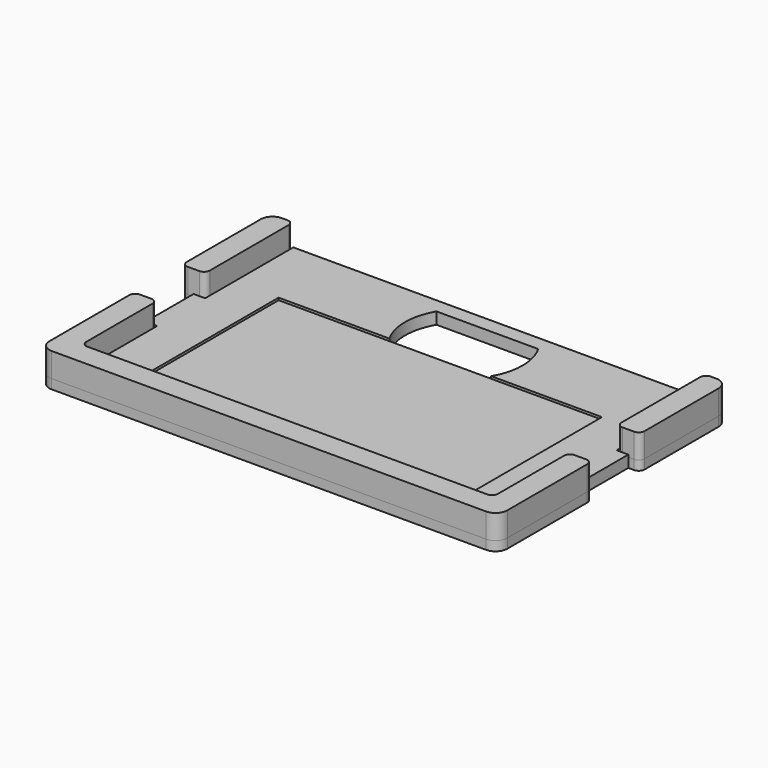
from build123d import *

# Parameters (mm, degrees)
F0_R     = 1.25
F0_W     = 2.5
F0_H     = 12.954
F0_W_2   = 69.85
F0_H_2   = 41.275
F1_DEPTH = 2.54
F2_DEPTH = 4.7625
F3_DEPTH = 0.5
F4_DEPTH = 0.5
F5_DEPTH = 3
F6_R     = 2.54
F6_2_R   = 2.54
F6_3_R   = 2.54
F6_4_R   = 2.54
F7_R     = 1.27
F7_2_R   = 1.27
F7_3_R   = 1.27
F7_4_R   = 1.27
F9_DEPTH = 2.541


with BuildPart() as f1:
    # F0 (on Top) → F1 (new body)
    with BuildSketch(Plane.XY):
        Polygon((44.45, 4.779), (44.45, 28.575), (-44.45, 28.575), (-44.45, 4.779), (-44.45, -8.175), (-44.45, -28.575), (-34.925, -28.575), (-34.925, 12.7), (34.925, 12.7), (34.925, -28.575), (44.45, -28.575), (44.45, -8.175), align=None)
        Polygon((-44.45, 4.779), (-44.45, 28.575), (-49.45, 28.575), (-49.45, 4.779), (-46.95, 4.779), align=None)
        with Locations((-46.95, 20.955)):
            Circle(F0_R, mode=Mode.SUBTRACT)
        Polygon((46.95, -8.175), (44.45, -8.175), (44.45, -28.575), (34.925, -28.575), (-34.925, -28.575), (-44.45, -28.575), (-44.45, -8.175), (-46.95, -8.175), (-49.45, -8.175), (-49.45, -33.575), (49.45, -33.575), (49.45, -8.175), align=None)
        with Locations((-46.95, -15.795)):
            Circle(F0_R, mode=Mode.SUBTRACT)
        with Locations((0, -31.075)):
            Circle(F0_R, mode=Mode.SUBTRACT)
        with Locations((46.95, -15.795)):
            Circle(F0_R, mode=Mode.SUBTRACT)
        with Locations((-45.7, -1.698)):
            Rectangle(F0_W, F0_H)
        with Locations((45.7, -1.698)):
            Rectangle(F0_W, F0_H)
        Polygon((49.45, 28.575), (44.45, 28.575), (44.45, 4.779), (46.95, 4.779), (49.45, 4.779), align=None)
        with Locations((46.95, 20.955)):
            Circle(F0_R, mode=Mode.SUBTRACT)
        with Locations((0, -7.9375)):
            Rectangle(F0_W_2, F0_H_2)
    extrude(amount=-F1_DEPTH)

    # F0 (on Top) → F3 (cut)
    with BuildSketch(Plane.XY):
        with Locations((0, -7.9375)):
            Rectangle(F0_W_2, F0_H_2)
        Polygon((46.95, -8.175), (44.45, -8.175), (44.45, -28.575), (34.925, -28.575), (-34.925, -28.575), (-44.45, -28.575), (-44.45, -8.175), (-46.95, -8.175), (-49.45, -8.175), (-49.45, -33.575), (49.45, -33.575), (49.45, -8.175), align=None)
        with Locations((-46.95, -15.795)):
            Circle(F0_R, mode=Mode.SUBTRACT)
        with Locations((0, -31.075)):
            Circle(F0_R, mode=Mode.SUBTRACT)
        with Locations((46.95, -15.795)):
            Circle(F0_R, mode=Mode.SUBTRACT)
        Polygon((49.45, 28.575), (44.45, 28.575), (44.45, 4.779), (46.95, 4.779), (49.45, 4.779), align=None)
        with Locations((46.95, 20.955)):
            Circle(F0_R, mode=Mode.SUBTRACT)
        Polygon((-44.45, 4.779), (-44.45, 28.575), (-49.45, 28.575), (-49.45, 4.779), (-46.95, 4.779), align=None)
        with Locations((-46.95, 20.955)):
            Circle(F0_R, mode=Mode.SUBTRACT)
    extrude(amount=-F3_DEPTH, mode=Mode.SUBTRACT)

    # F6
    f6_edges = [f1.edges().sort_by_distance(p)[0] for p in [
        (-49.45, -33.575, -1.52),
        (-49.45, 28.575, -1.52),
        (49.45, -33.575, -1.52),
        (49.45, 28.575, -1.52),
    ]]
    fillet(f6_edges, radius=F6_R)

    # F7
    f7_edges = [f1.edges().sort_by_distance(p)[0] for p in [
        (49.45, 4.779, -1.52),
        (49.45, -8.175, -1.52),
        (-49.45, 4.779, -1.52),
        (-49.45, -8.175, -1.52),
        (44.45, -28.575, -0.25),
        (-44.45, -28.575, -0.25),
    ]]
    fillet(f7_edges, radius=F7_R)

    # F8 (on face) → F9 (cut, through all)
    with BuildSketch(Plane.XY):
        with BuildLine():
            ThreePointArc((10.9985226281, 12.7), (12.2672579939, 15.7629981272), (12.7, 19.05))
            ThreePointArc((12.7, 19.05), (12.2672579939, 22.3370018728), (10.9985226281, 25.4))
            Line((10.9985226281, 25.4), (-10.9985226281, 25.4))
            ThreePointArc((-10.9985226281, 25.4), (-12.7, 19.05), (-10.9985226281, 12.7))
            Line((-10.9985226281, 12.7), (10.9985226281, 12.7))
        make_face()
    extrude(amount=-F9_DEPTH, mode=Mode.SUBTRACT)


with BuildPart() as f2:
    # F0 (on Top) → F2 (new body)
    with BuildSketch(Plane.XY):
        Polygon((-44.45, 4.779), (-44.45, 28.575), (-49.45, 28.575), (-49.45, 4.779), (-46.95, 4.779), align=None)
        with Locations((-46.95, 20.955)):
            Circle(F0_R, mode=Mode.SUBTRACT)
        with Locations((-46.95, 20.955)):
            Circle(F0_R)
    extrude(amount=F2_DEPTH)

    # F4#3 (add): a face of the model
    f4_3_faces = [f2.faces().sort_by_distance(p)[0] for p in [
        (-46.95, 16.677, 0),
    ]]
    extrude(f4_3_faces, amount=F4_DEPTH)


with BuildPart() as f2b:
    # F0 (on Top) → F2, piece 2 (new body)
    with BuildSketch(Plane.XY):
        Polygon((49.45, 28.575), (44.45, 28.575), (44.45, 4.779), (46.95, 4.779), (49.45, 4.779), align=None)
        with Locations((46.95, 20.955)):
            Circle(F0_R, mode=Mode.SUBTRACT)
        with Locations((46.95, 20.955)):
            Circle(F0_R)
    extrude(amount=F2_DEPTH)

    # F4#2 (add): a face of the model
    f4_2_faces = [f2b.faces().sort_by_distance(p)[0] for p in [
        (46.95, 16.677, 0),
    ]]
    extrude(f4_2_faces, amount=F4_DEPTH)


with BuildPart() as f2c:
    # F0 (on Top) → F2, piece 3 (new body)
    with BuildSketch(Plane.XY):
        Polygon((46.95, -8.175), (44.45, -8.175), (44.45, -28.575), (34.925, -28.575), (-34.925, -28.575), (-44.45, -28.575), (-44.45, -8.175), (-46.95, -8.175), (-49.45, -8.175), (-49.45, -33.575), (49.45, -33.575), (49.45, -8.175), align=None)
        with Locations((-46.95, -15.795)):
            Circle(F0_R, mode=Mode.SUBTRACT)
        with Locations((0, -31.075)):
            Circle(F0_R, mode=Mode.SUBTRACT)
        with Locations((46.95, -15.795)):
            Circle(F0_R, mode=Mode.SUBTRACT)
        with Locations((-46.95, -15.795)):
            Circle(F0_R)
        with Locations((0, -31.075)):
            Circle(F0_R)
        with Locations((46.95, -15.795)):
            Circle(F0_R)
    extrude(amount=F2_DEPTH)

    # F4 (add): a face of the model
    f4_faces = [f2c.faces().sort_by_distance(p)[0] for p in [
        (45.4710959798, -18.375, 0),
    ]]
    extrude(f4_faces, amount=F4_DEPTH)


with BuildPart() as f5_tool:
    # F0 (on Top) → F5 (new body, symmetric)
    with BuildSketch(Plane.XY):
        with Locations((-46.95, -15.795)):
            Circle(F0_R)
        with Locations((0, -31.075)):
            Circle(F0_R)
        with Locations((46.95, -15.795)):
            Circle(F0_R)
        with Locations((46.95, 20.955)):
            Circle(F0_R)
        with Locations((-46.95, 20.955)):
            Circle(F0_R)
    extrude(amount=F5_DEPTH, both=True)


with BuildPart() as f2_1:
    add(f2.part)

    # F5: cut by f5_tool
    add(f5_tool.part, mode=Mode.SUBTRACT)

    # F6#2
    f6_2_edges = [f2_1.edges().sort_by_distance(p)[0] for p in [
        (-49.45, 28.575, 2.13125),
    ]]
    fillet(f6_2_edges, radius=F6_2_R)

    # F7#2
    f7_2_edges = [f2_1.edges().sort_by_distance(p)[0] for p in [
        (-49.45, 4.779, 2.13125),
        (-44.45, 4.779, 2.13125),
        (-44.45, 28.575, 2.13125),
    ]]
    fillet(f7_2_edges, radius=F7_2_R)


with BuildPart() as f2b_1:
    add(f2b.part)

    # F5: cut by f5_tool
    add(f5_tool.part, mode=Mode.SUBTRACT)

    # F6#3
    f6_3_edges = [f2b_1.edges().sort_by_distance(p)[0] for p in [
        (49.45, 28.575, 2.13125),
    ]]
    fillet(f6_3_edges, radius=F6_3_R)

    # F7#3
    f7_3_edges = [f2b_1.edges().sort_by_distance(p)[0] for p in [
        (49.45, 4.779, 2.13125),
        (44.45, 4.779, 2.13125),
        (44.45, 28.575, 2.13125),
    ]]
    fillet(f7_3_edges, radius=F7_3_R)


with BuildPart() as f2c_1:
    add(f2c.part)

    # F5: cut by f5_tool
    add(f5_tool.part, mode=Mode.SUBTRACT)

    # F6#4
    f6_4_edges = [f2c_1.edges().sort_by_distance(p)[0] for p in [
        (-49.45, -33.575, 2.13125),
        (49.45, -33.575, 2.13125),
    ]]
    fillet(f6_4_edges, radius=F6_4_R)

    # F7#4
    f7_4_edges = [f2c_1.edges().sort_by_distance(p)[0] for p in [
        (49.45, -8.175, 2.13125),
        (-49.45, -8.175, 2.13125),
        (-44.45, -8.175, 2.13125),
        (44.45, -8.175, 2.13125),
        (-44.45, -28.575, 2.13125),
        (44.45, -28.575, 2.13125),
    ]]
    fillet(f7_4_edges, radius=F7_4_R)


solid = Compound([f1.part, f2_1.part, f2b_1.part, f2c_1.part])
